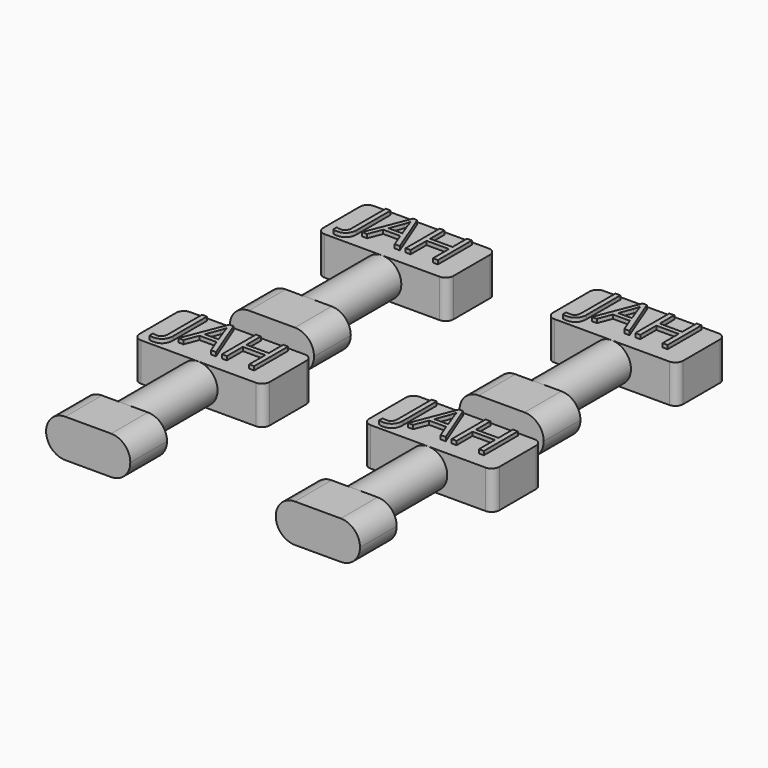
from build123d import *

# Parameters (mm, degrees)
F0_W         = 8
F0_H         = 17
F1_DEPTH     = 5
F2_R         = 2.5
F3_DEPTH     = 12
F5_DEPTH     = 6
F6_ANGLE     = -90
F7_TEXT_SIZE = 7.7726409978
F8_DEPTH     = 0.5
F9_R         = 1


# Not quite as in the source:
# - Text() gives the source's letters only with a copy of the font that has no kerning and outlines rounded to 1/6400 em; it was checked with that copy


with BuildPart() as f1:
    # F0 (on Top) → F1 (new body)
    with BuildSketch(Plane.XY):
        with Locations((8.5, 0)):
            Rectangle(F0_W, F0_H)
    extrude(amount=F1_DEPTH)

    # F2 (on face) → F3 (join)
    with BuildSketch(Plane(origin=(4.5, 0, 0), x_dir=(0, -1, 0), z_dir=(-1, 0, 0))):
        with Locations((0, 2.5)):
            Circle(F2_R)
    extrude(amount=F3_DEPTH)

    # F4 (on face) → F5 (join)
    with BuildSketch(Plane(origin=(-7.5, 0, 0), x_dir=(0, -1, 0), z_dir=(-1, 0, 0))):
        with BuildLine():
            ThreePointArc((-3, 0), (-1.232233047, 0.732233047), (-0.5, 2.5))
            ThreePointArc((-0.5, 2.5), (-1.232233047, 4.267766953), (-3, 5))
            ThreePointArc((-3, 5), (-5.5, 2.5), (-3, 0))
        make_face()
        with BuildLine():
            ThreePointArc((-3, 5), (-1.232233047, 4.267766953), (-0.5, 2.5))
            ThreePointArc((-0.5, 2.5), (-1.232233047, 0.732233047), (-3, 0))
            Line((-3, 0), (3, 0))
            ThreePointArc((3, 0), (0.5, 2.5), (3, 5))
            Line((3, 5), (-3, 5))
        make_face()
        with BuildLine():
            ThreePointArc((5.5, 2.5), (4.767766953, 4.267766953), (3, 5))
            ThreePointArc((3, 5), (0.5, 2.5), (3, 0))
            ThreePointArc((3, 0), (4.767766953, 0.732233047), (5.5, 2.5))
        make_face()
    extrude(amount=F5_DEPTH)


with BuildPart() as f1_1:
    # F6: moved
    add(f1.part.rotate(Axis((12.5, -8.5, 2.5), (0, 0, -1)), F6_ANGLE))

    # F7 (on face) → F8 (join)
    with BuildSketch(Plane.XY.offset(5)):
        with Locations((-2.2885523572, -14.5)):
            Text('JAH', F7_TEXT_SIZE, font='Open Sans', text_align=(TextAlign.LEFT, TextAlign.BOTTOM))
    extrude(amount=F8_DEPTH)

    # F9
    f9_edges = [f1_1.edges().sort_by_distance(p)[0] for p in [
        (-4.5, -8.5, 2.5),
        (-4.5, -16.5, 2.5),
        (12.5, -8.5, 2.5),
        (12.5, -16.5, 2.5),
    ]]
    fillet(f9_edges, radius=F9_R)


with BuildPart() as f10_1:
    # F10: copy of F1
    add(f1_1.part.moved(Location((30, 0, 0))))


with BuildPart() as f11_1:
    # F11: copy of F1
    add(f1_1.part.moved(Location((0, 30, 0))))


with BuildPart() as f12_1:
    # F12: copy of F1
    add(f1_1.part.moved(Location((30, 30, 0))))


solid = Compound([f1_1.part, f10_1.part, f11_1.part, f12_1.part])
